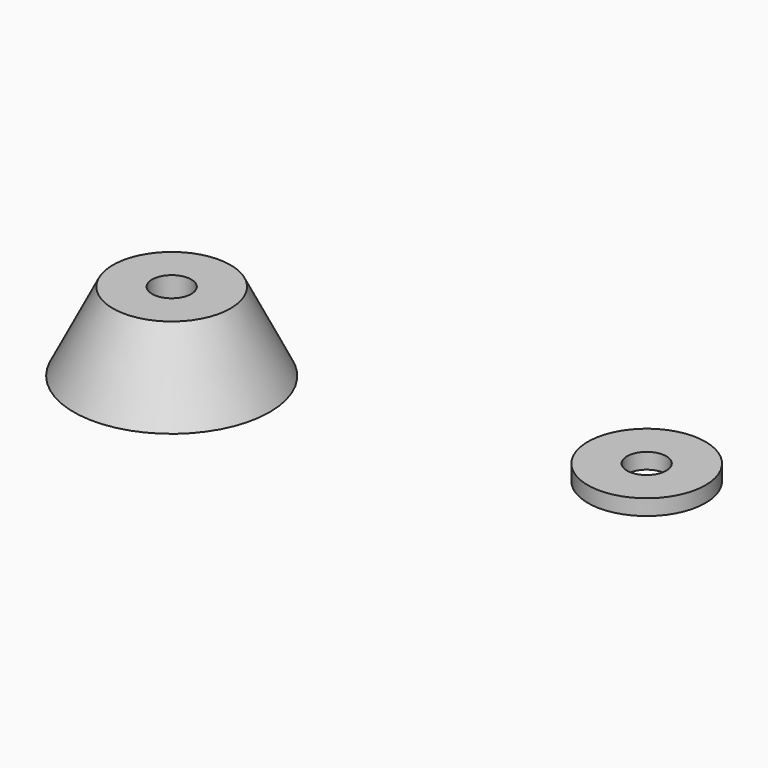
from build123d import *

# Parameters (mm, degrees)
F0_R     = 12.5
F0_R_2   = 2.5
F1_DEPTH = 10
F0_R_3   = 7.5
F2_DEPTH = 2
F3_SIZE2 = 9.99999
F3_SIZE  = 4.99999


# Not quite as in the source:
# - a fillet or chamfer is up to 0.001 mm smaller than in the source, because OpenCascade refuses the exact size


with BuildPart() as f1:
    # F0 (on Top) → F1 (new body)
    with BuildSketch(Plane.XY):
        with Locations((-34.0288244188, 0)):
            Circle(F0_R)
        with Locations((-34.0288244188, 0)):
            Circle(F0_R_2, mode=Mode.SUBTRACT)
    extrude(amount=F1_DEPTH)

    # F3 (size 5 and 10 in the source; OpenCascade refuses exactly that, so slightly less here)
    f3_edges = [f1.edges().sort_by_distance(p)[0] for p in [
        (-46.528824, 0, 10),
    ]]
    f3_side = f1.faces().sort_by_distance((-46.175271, 0, 10))[0]
    chamfer(f3_edges, length=F3_SIZE, length2=F3_SIZE2, reference=f3_side)


with BuildPart() as f2:
    # F0 (on Top) → F2 (new body)
    with BuildSketch(Plane.XY):
        with Locations((17.0663259923, 11.785466224)):
            Circle(F0_R_3)
        with Locations((17.0663259923, 11.785466224)):
            Circle(F0_R_2, mode=Mode.SUBTRACT)
    extrude(amount=F2_DEPTH)


solid = Compound([f1.part, f2.part])
